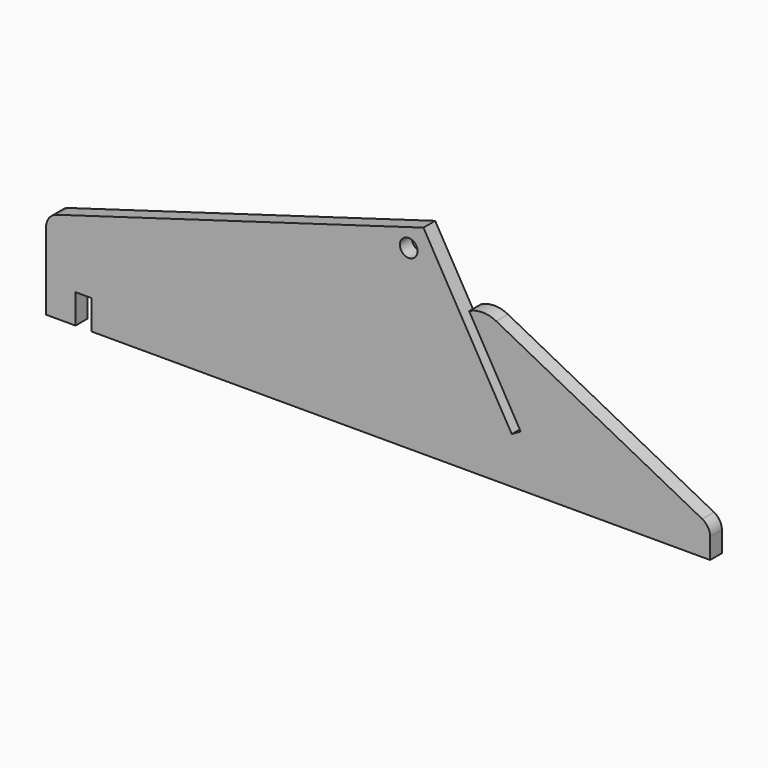
from build123d import *

# Parameters (mm, degrees)
F0_R        = 3
F1_DEPTH    = 5
F2_T1_DEPTH = 32.3482938807
F3_R        = 5


# Not quite as in the source:
# - a fillet or chamfer that OpenCascade refuses, or shapes differently, is made with other operations: its cross-section is extruded or revolved along the edge and cut away or added


with BuildPart() as f1:
    # F0 (on Front) → F1 (new body)
    with BuildSketch(Plane.XZ):
        Polygon((0, 30), (0, 0), (10, 0), (10, 10), (15.5, 10), (15.5, 0), (165.5, 0), (165.5, 20), (148, 50.3108891325), (143.6698729811, 47.8108891325), (161.1698729811, 17.5), (158.1387840678, 15.75), (128.1387840678, 67.7115242271), align=None)
        with Locations((123.1387840678, 60)):
            Circle(F0_R, mode=Mode.SUBTRACT)
        Polygon((165.5, 20), (165.5, 0), (225.5, 0), (225.5, 10), (148, 50.3108891325), align=None)
    extrude(amount=F1_DEPTH)

    # F2: fillet of radius 10 on 1 edges, made by hand

    # F2_s2 → F2_t1 (cut)
    with BuildSketch(Plane.XZ.offset(-13.6741469404)):
        with BuildLine():
            ThreePointArc((152.8524940595, 47.7869104222), (148.2640985796, 48.9152185915), (143.6698729811, 47.8108891325))
            Line((143.6698729811, 47.8108891325), (148, 50.3108891325))
            Line((148, 50.3108891325), (152.8524940595, 47.7869104222))
        make_face()
    extrude(amount=F2_T1_DEPTH, mode=Mode.SUBTRACT)

    # F3
    f3_edges = [f1.edges().sort_by_distance(p)[0] for p in [
        (225.5, -2.5, 10),
        (0, -2.5, 30),
    ]]
    fillet(f3_edges, radius=F3_R)


solid = f1.part
